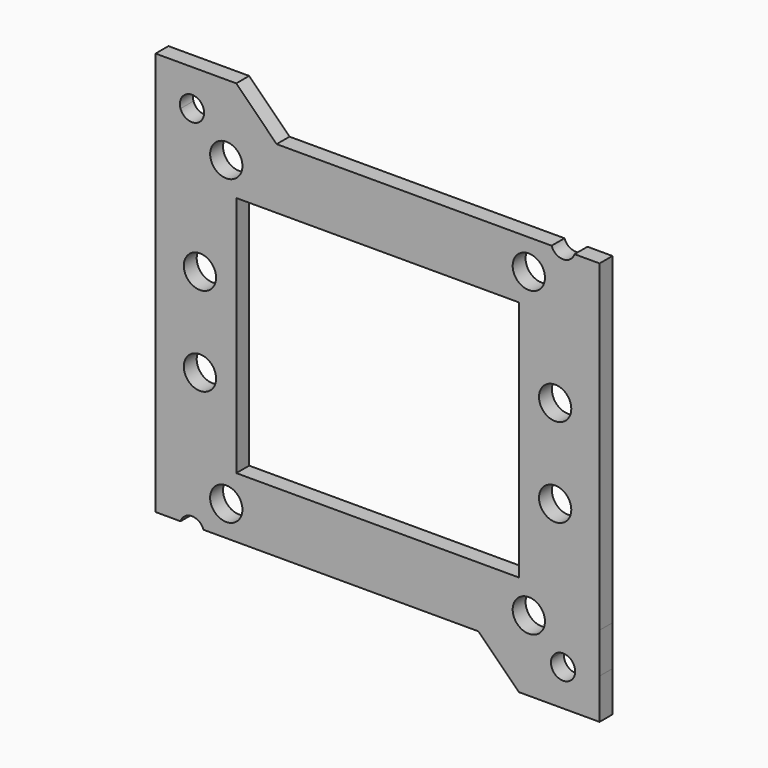
from build123d import *

# Parameters (mm, degrees)
F0_R     = 2
F1_DEPTH = 2


# Not quite as in the source:
# - ends of sketch curves that miss each other by under 0.0002 mm in the source are joined
# - a feature names something its author has since deleted; it is built from what else it names


with BuildPart() as f1:
    # F0 (on Front) → F1 (new body)
    with BuildSketch(Plane.XZ):
        with BuildLine():
            Line((21.5601722026, 22.5), (-12.5000000166, 22.5))
            Line((-12.5000000166, 22.5), (-5.0000000414, 15))
            Line((-5.0000000414, 15), (17.5, 15))
            Line((17.5, 15), (17.5, -7.5000001159))
            Line((17.5, -7.5000001159), (27.499999851, -17.5))
            Line((27.499999851, -17.5), (27.5, 22.5))
            Line((27.5, 22.5), (24.4017685746, 22.5))
            ThreePointArc((24.4017685746, 22.5), (22.9809703886, 21.4809703886), (21.5601722026, 22.5))
        make_face()
        with Locations((22, -5.5)):
            Circle(F0_R, mode=Mode.SUBTRACT)
        with Locations((22, 5.5)):
            Circle(F0_R, mode=Mode.SUBTRACT)
        with Locations((18.7383297014, 18.7383297014)):
            Circle(F0_R, mode=Mode.SUBTRACT)
        with BuildLine():
            Line((27.499999851, -17.5), (17.5, -7.5000001159))
            Line((17.5, -7.5000001159), (17.5, -15))
            Line((17.5, -15), (5, -15))
            Line((5, -15), (12.5, -22.5))
            Line((12.5, -22.5), (21.5601722026, -22.5))
            ThreePointArc((21.5601722026, -22.5), (22.9809703886, -21.4809703886), (24.4017685746, -22.5))
            Line((24.4017685746, -22.5), (27.5, -22.5))
            Line((27.5, -22.5), (27.499999851, -17.5))
        make_face()
        with Locations((18.7383297014, -18.7383297014)):
            Circle(F0_R, mode=Mode.SUBTRACT)
        with BuildLine():
            Line((21.5601722026, -22.5), (12.5, -22.5))
            Line((12.5, -22.5), (17.5, -27.5))
            Line((17.5, -27.5), (27.5, -27.5))
            Line((27.5, -27.5), (27.5, -22.5))
            Line((27.5, -22.5), (24.4017685746, -22.5))
            ThreePointArc((24.4017685746, -22.5), (24.461037495, -22.7372464453), (24.4809703886, -22.9809703886))
            ThreePointArc((24.4809703886, -22.9809703886), (22.7372464453, -24.461037495), (21.5601722026, -22.5))
        make_face()
        with BuildLine():
            Line((-17.5, 7.5), (-27.5, 17.5))
            Line((-27.5, 17.5), (-27.5, -22.5))
            Line((-27.5, -22.5), (-24.4017685746, -22.5))
            ThreePointArc((-24.4017685746, -22.5), (-22.9809703886, -21.4809703886), (-21.5601722026, -22.5))
            Line((-21.5601722026, -22.5), (12.5, -22.5))
            Line((12.5, -22.5), (5, -15))
            Line((5, -15), (-17.5, -15))
            Line((-17.5, -15), (-17.5, 7.5))
        make_face()
        with Locations((-18.7383297014, -18.7383297014)):
            Circle(F0_R, mode=Mode.SUBTRACT)
        with Locations((-22, -5.5)):
            Circle(F0_R, mode=Mode.SUBTRACT)
        with Locations((-22, 5.5)):
            Circle(F0_R, mode=Mode.SUBTRACT)
        with BuildLine():
            ThreePointArc((-21.5601722026, 22.5), (-22.9809703886, 21.4809703886), (-24.4017685746, 22.5))
            Line((-24.4017685746, 22.5), (-27.5, 22.5))
            Line((-27.5, 22.5), (-27.5, 17.5))
            Line((-27.5, 17.5), (-17.5, 7.5))
            Line((-17.5, 7.5), (-17.5, 15))
            Line((-17.5, 15), (-5.0000000414, 15))
            Line((-5.0000000414, 15), (-12.5000000166, 22.5))
            Line((-12.5000000166, 22.5), (-21.5601722026, 22.5))
        make_face()
        with Locations((-18.7383297014, 18.7383297014)):
            Circle(F0_R, mode=Mode.SUBTRACT)
        with BuildLine():
            ThreePointArc((-24.4017685746, 22.5), (-23.2246943318, 24.461037495), (-21.4809703886, 22.9809703886))
            ThreePointArc((-21.4809703886, 22.9809703886), (-21.5009032821, 22.7372464453), (-21.5601722026, 22.5))
            Line((-21.5601722026, 22.5), (-12.5000000166, 22.5))
            Line((-12.5000000166, 22.5), (-17.5, 27.5))
            Line((-17.5, 27.5), (-27.5, 27.5))
            Line((-27.5, 27.5), (-27.5, 22.5))
            Line((-27.5, 22.5), (-24.4017685746, 22.5))
        make_face()
    extrude(amount=F1_DEPTH)


solid = f1.part
